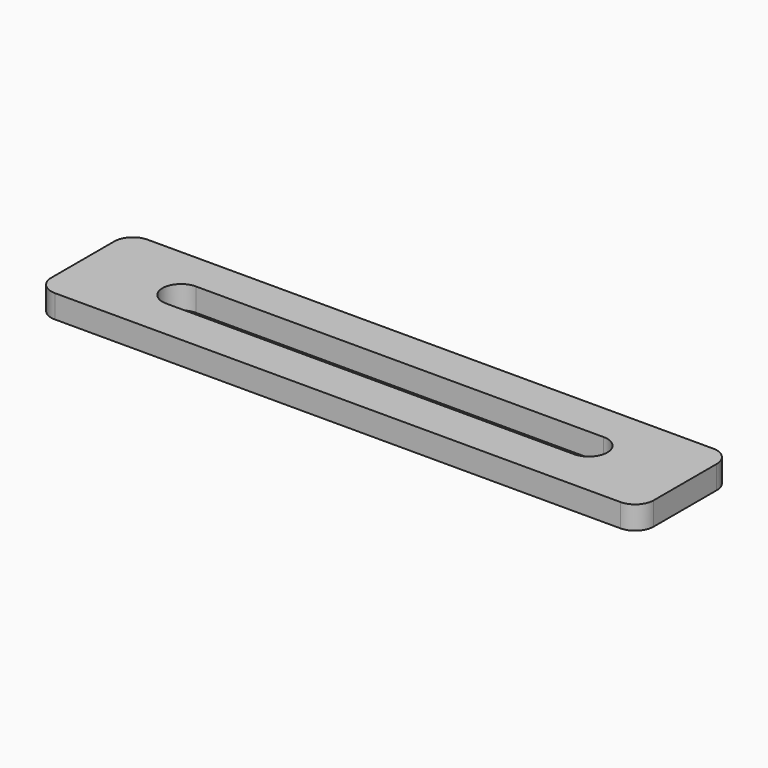
from build123d import *

# Parameters (mm, degrees)
F1_W     = 165.1
F1_H     = 31.75
F2_DEPTH = 6.35
F3_R     = 5.08


# Not quite as in the source:
# - a variable given as a bare number and used for a length is read in inches; the dataset says mm whatever the document's units were


with BuildPart() as f2:
    # F1 (on Top) → F2 (new body)
    with BuildSketch(Plane.XY):
        with Locations((0, -0.3175)):
            Rectangle(F1_W, F1_H)
        with BuildLine():
            ThreePointArc((-55.88, -5.08), (-60.96, 0), (-55.88, 5.08))
            Line((-55.88, 5.08), (0, 5.08))
            Line((0, 5.08), (55.88, 5.08))
            ThreePointArc((55.88, 5.08), (60.96, 0), (55.88, -5.08))
            Line((55.88, -5.08), (0, -5.08))
            Line((0, -5.08), (-55.88, -5.08))
        make_face(mode=Mode.SUBTRACT)
    extrude(amount=F2_DEPTH)

    # F3
    f3_edges = [f2.edges().sort_by_distance(p)[0] for p in [
        (-82.55, 15.5575, 3.175),
        (-82.55, -16.1925, 3.175),
        (82.55, 15.5575, 3.175),
        (82.55, -16.1925, 3.175),
    ]]
    fillet(f3_edges, radius=F3_R)


solid = f2.part
